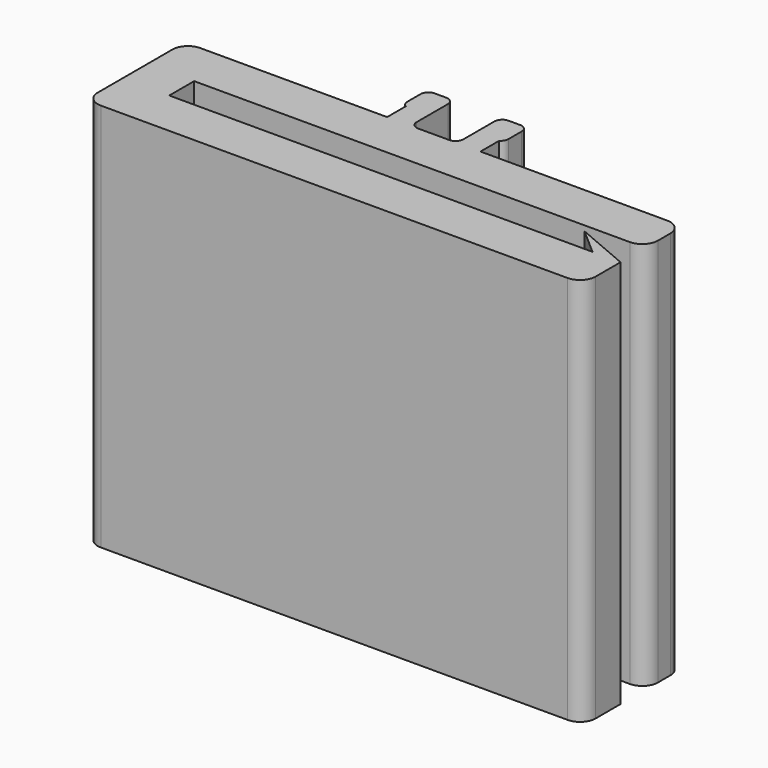
from build123d import *

# Parameters (mm, degrees)
F1_DEPTH     = 25
F2_R         = 1
F3_T1_DEPTH  = 25
F3_T3_DEPTH  = 25
F3_T5_DEPTH  = 27.1650635095
F3_T7_DEPTH  = 27.5
F3_T9_DEPTH  = 27.5
F3_T11_DEPTH = 27.5
F3_T13_DEPTH = 27.5
F3_T15_DEPTH = 27.1650635095


# Not quite as in the source:
# - a fillet or chamfer that OpenCascade refuses, or shapes differently, is made with other operations: its cross-section is extruded or revolved along the edge and cut away or added


with BuildPart() as f1:
    # F0 (on Top) → F1 (new body)
    with BuildSketch(Plane.XY):
        Polygon((0, 8), (0, 0), (32, 0), (32, 3), (30.2, 3), (3, 3), (3, 5), (32, 5), (32, 8), (19, 8), (19, 9.5), (19.25, 9.5), (19.25, 11.5), (17.5, 11.5), (17.5, 8), (14.5, 8), (14.5, 11.5), (12.75, 11.5), (12.75, 9.5), (13, 9.5), (13, 8), align=None)
        Polygon((30.2, 3), (32, 3), (28.4834179878, 4.5), align=None)
    extrude(amount=F1_DEPTH)

    # F2
    f2_edges = [f1.edges().sort_by_distance(p)[0] for p in [
        (32, 8, 12.5),
        (32, 5, 12.5),
        (32, 0, 12.5),
        (0, 0, 12.5),
        (0, 8, 12.5),
    ]]
    fillet(f2_edges, radius=F2_R)

    # F3: fillet of radius 0.5 on 8 edges, made by hand

    # F3_s2 → F3_t1 (join)
    with BuildSketch(Plane.XY):
        with BuildLine():
            ThreePointArc((14.5, 8.5), (14.6464466094, 8.1464466094), (15, 8))
            Line((15, 8), (14.5, 8))
            Line((14.5, 8), (14.5, 8.5))
        make_face()
    extrude(amount=F3_T1_DEPTH)

    # F3_s4 → F3_t3 (join)
    with BuildSketch(Plane.XY):
        with BuildLine():
            ThreePointArc((17, 8), (17.3535533906, 8.1464466094), (17.5, 8.5))
            Line((17.5, 8.5), (17.5, 8))
            Line((17.5, 8), (17, 8))
        make_face()
    extrude(amount=F3_T3_DEPTH)

    # F3_s6 → F3_t5 (cut)
    with BuildSketch(Plane.XY.offset(-1.0825317547)):
        with BuildLine():
            ThreePointArc((12.75, 9.9330127019), (12.8169872981, 9.6830127019), (13, 9.5))
            Line((13, 9.5), (12.75, 9.5))
            Line((12.75, 9.5), (12.75, 9.9330127019))
        make_face()
    extrude(amount=F3_T5_DEPTH, mode=Mode.SUBTRACT)

    # F3_s8 → F3_t7 (cut)
    with BuildSketch(Plane.XY.offset(-1.25)):
        with BuildLine():
            ThreePointArc((12.75, 11), (12.8964466094, 11.3535533906), (13.25, 11.5))
            Line((13.25, 11.5), (12.75, 11.5))
            Line((12.75, 11.5), (12.75, 11))
        make_face()
    extrude(amount=F3_T7_DEPTH, mode=Mode.SUBTRACT)

    # F3_s10 → F3_t9 (cut)
    with BuildSketch(Plane.XY.offset(-1.25)):
        with BuildLine():
            ThreePointArc((14, 11.5), (14.3535533906, 11.3535533906), (14.5, 11))
            Line((14.5, 11), (14.5, 11.5))
            Line((14.5, 11.5), (14, 11.5))
        make_face()
    extrude(amount=F3_T9_DEPTH, mode=Mode.SUBTRACT)

    # F3_s12 → F3_t11 (cut)
    with BuildSketch(Plane.XY.offset(-1.25)):
        with BuildLine():
            ThreePointArc((17.5, 11), (17.6464466094, 11.3535533906), (18, 11.5))
            Line((18, 11.5), (17.5, 11.5))
            Line((17.5, 11.5), (17.5, 11))
        make_face()
    extrude(amount=F3_T11_DEPTH, mode=Mode.SUBTRACT)

    # F3_s14 → F3_t13 (cut)
    with BuildSketch(Plane.XY.offset(-1.25)):
        with BuildLine():
            ThreePointArc((18.75, 11.5), (19.1035533906, 11.3535533906), (19.25, 11))
            Line((19.25, 11), (19.25, 11.5))
            Line((19.25, 11.5), (18.75, 11.5))
        make_face()
    extrude(amount=F3_T13_DEPTH, mode=Mode.SUBTRACT)

    # F3_s16 → F3_t15 (cut)
    with BuildSketch(Plane.XY.offset(-1.0825317547)):
        with BuildLine():
            ThreePointArc((19.25, 9.9330127019), (19.1830127019, 9.6830127019), (19, 9.5))
            Line((19, 9.5), (19.25, 9.5))
            Line((19.25, 9.5), (19.25, 9.9330127019))
        make_face()
    extrude(amount=F3_T15_DEPTH, mode=Mode.SUBTRACT)


solid = f1.part
